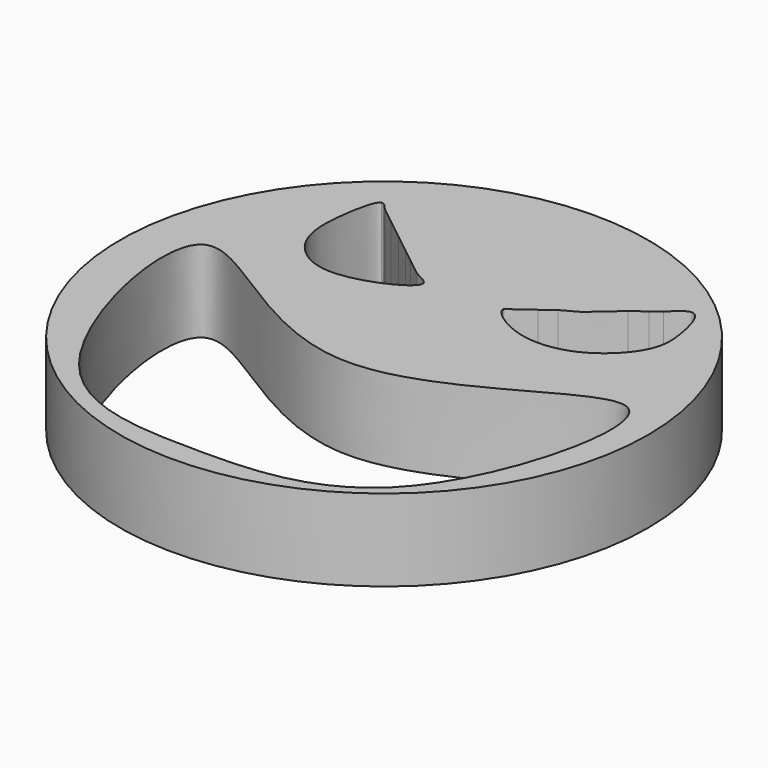
from build123d import *

# Parameters (mm, degrees)
F0_R     = 81.902918293
F1_DEPTH = 25.4


with BuildPart() as f1:
    # F0 (on Top) → F1 (new body)
    with BuildSketch(Plane.XY):
        Circle(F0_R)
        with BuildLine():
            add(Edge.make_bspline(
                [(-64.7033080459, 10.6473797932), (-55.638691326, 16.2235461657), (-0.5013684948, -46.3821262938), (88.1133259334, 43.339149836), (61.4765252175, -73.4087770429), (-0.1257711411, -75.3164533915), (-57.1020292766, -72.3904873582), (-73.6575101256, 5.1391358077), (-64.7033080459, 10.6473797932)],
                knots=[0, 0, 0, 0, 0.1735094926, 0.3511757019, 0.519828612, 0.6769418156, 0.8286039986, 1, 1, 1, 1], degree=3))
        make_face(mode=Mode.SUBTRACT)
        with BuildLine():
            add(Edge.make_bspline(
                [(-10.3197693825, 27.6831854135), (-10.7546762642, 24.6549609474), (-32.7110043658, 14.0295047318), (-48.8070708673, 26.7191397879), (-48.7153193022, 42.2672541357), (-46.2129546559, 54.4217754372), (-44.7189956903, 54.8749603331)],
                knots=[0, 0, 0, 0, 0.1402195568, 0.264912908, 0.383777657, 0.484604884, 0.484604884, 0.484604884, 0.484604884], degree=3))
            add(Edge.make_bspline(
                [(-44.7189956903, 54.8749603331), (-43.8655444042, 55.1338504641), (-42.8993390105, 53.7201742756), (-41.7464575259, 52.525239209)],
                knots=[0.484604884, 0.484604884, 0.484604884, 0.484604884, 0.542204275, 0.542204275, 0.542204275, 0.542204275], degree=3))
            Line((-41.7464575259, 52.525239209), (-36.4907558108, 48.3707312906))
            add(Edge.make_bspline(
                [(-36.4907558108, 48.3707312906), (-34.5004466095, 46.9114950565), (-32.5139801247, 45.2674795506), (-30.4707956879, 43.6120951742)],
                knots=[0.6187938265, 0.6187938265, 0.6187938265, 0.6187938265, 0.7007630798, 0.7007630798, 0.7007630798, 0.7007630798], degree=3))
            Line((-30.4707956879, 43.6120951742), (-24.5679702911, 38.9460512887))
            add(Edge.make_bspline(
                [(-24.5679702911, 38.9460512887), (-23.0462694735, 37.7828890396), (-21.7230970705, 36.8152719658), (-20.3530360137, 35.6142454177)],
                knots=[0.7819309481, 0.7819309481, 0.7819309481, 0.7819309481, 0.850519175, 0.850519175, 0.850519175, 0.850519175], degree=3))
            Line((-20.3530360137, 35.6142454177), (-14.8534622354, 31.2669624005))
            add(Edge.make_bspline(
                [(-14.8534622354, 31.2669624005), (-12.7575228708, 30.0875918291), (-10.0991376837, 29.2194276214), (-10.3197693825, 27.6831854135)],
                knots=[0.9288655105, 0.9288655105, 0.9288655105, 0.9288655105, 1, 1, 1, 1], degree=3))
        make_face(mode=Mode.SUBTRACT)
        with BuildLine():
            add(Edge.make_bspline(
                [(20.0402461774, 34.6573553744), (19.0855216744, 33.9199072149), (17.4015863072, 32.7935603855), (15.6728127348, 31.0543564349), (13.3584732412, 30.3603178638), (13.2682733238, 29.5815523714)],
                knots=[0.869222989, 0.869222989, 0.869222989, 0.869222989, 0.9159771846, 0.9577752247, 1, 1, 1, 1], degree=3))
            add(Edge.make_bspline(
                [(23.9551238818, 37.5916772387), (22.4871119125, 36.6865231729), (21.214072016, 35.5640417552), (20.0402461774, 34.6573553744)],
                knots=[0.8117390943, 0.8117390943, 0.8117390943, 0.8117390943, 0.869222989, 0.869222989, 0.869222989, 0.869222989], degree=3))
            add(Edge.make_bspline(
                [(37.5341082285, 47.7695457881), (36.2480528135, 46.7505662168), (32.5629459388, 43.6976408534), (29.262387548, 40.0600353259), (25.5221471778, 38.5578801969), (23.9551238818, 37.5916772387)],
                knots=[0.6461857755, 0.6461857755, 0.6461857755, 0.6461857755, 0.6834655967, 0.750378149, 0.8117390943, 0.8117390943, 0.8117390943, 0.8117390943], degree=3))
            add(Edge.make_bspline(
                [(41.6016501152, 50.8182941765), (40.5640970851, 50.102162609), (39.0723272323, 48.9883219955), (37.5341082285, 47.7695457881)],
                knots=[0.6015963056, 0.6015963056, 0.6015963056, 0.6015963056, 0.6461857755, 0.6461857755, 0.6461857755, 0.6461857755], degree=3))
            Line((41.6016501152, 50.8182941765), (44.3913824856, 52.9092848301))
            add(Edge.make_bspline(
                [(13.2682733238, 29.5815523714), (13.0796071411, 27.9526516269), (23.3956142868, 19.9149627224), (42.3360455892, 21.1472231964), (55.603881243, 34.9274274397), (55.5617796072, 45.6068310596), (51.5625129671, 60.7711012443), (45.9215093945, 54.3448631124), (44.3913824856, 52.9092848301)],
                knots=[0, 0, 0, 0, 0.0883192291, 0.202241682, 0.3095000963, 0.3969770332, 0.4836397483, 0.5530709914, 0.5530709914, 0.5530709914, 0.5530709914], degree=3))
        make_face(mode=Mode.SUBTRACT)
        with BuildLine():
            add(Edge.make_bspline(
                [(23.9551238818, 37.5916772387), (22.4871119125, 36.6865231729), (21.214072016, 35.5640417552), (20.0402461774, 34.6573553744)],
                knots=[0.8117390943, 0.8117390943, 0.8117390943, 0.8117390943, 0.869222989, 0.869222989, 0.869222989, 0.869222989], degree=3))
            Line((20.0402461774, 34.6573553744), (23.9551238818, 37.5916772387))
        make_face()
    extrude(amount=F1_DEPTH)


solid = f1.part
